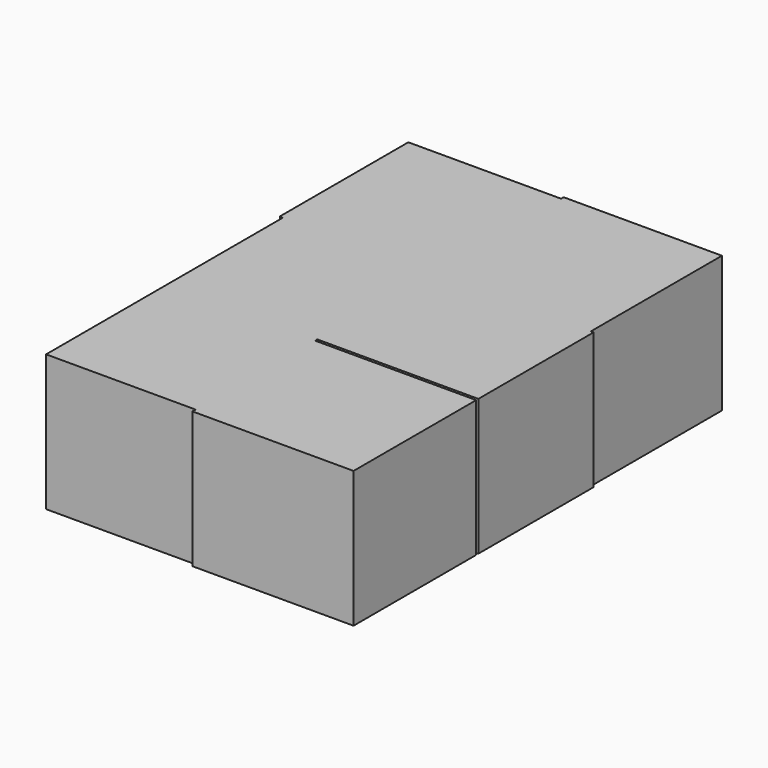
from build123d import *

# Parameters (mm, degrees)
F0_W     = 39.7309437394
F0_H     = 35.8594581485
F0_H_2   = 34.1520495713
F0_W_2   = 39.8523285985
F1_DEPTH = 25.4
F2_W     = 39.7309437394
F2_H     = 34.1520495713
F3_DEPTH = 25.4
F5_W     = 33.1652238965
F5_H     = 31.9460257888
F6_DEPTH = 30.226


with BuildPart() as f1:
    # F0 (on Top) → F1 (new body)
    with BuildSketch(Plane.XY):
        with Locations((-19.8654718697, 17.9297290742)):
            Rectangle(F0_W, F0_H)
        with Locations((-19.8654718697, -17.0760247856)):
            Rectangle(F0_W, F0_H_2)
        with Locations((19.9261642992, 17.9297290742)):
            Rectangle(F0_W_2, F0_H)
    extrude(amount=F1_DEPTH)

    # F2 (on face) → F3 (join)
    with BuildSketch(Plane.XY.offset(25.4)):
        with Locations((-19.8654718697, -17.0760247856)):
            Rectangle(F2_W, F2_H)
    extrude(amount=F3_DEPTH)


with BuildPart() as f6:
    # F5 (on Top) → F6 (new body)
    with BuildSketch(Plane.XY):
        with Locations((-16.5826119483, -15.9730128944)):
            Rectangle(F5_W, F5_H)
        Polygon((-33.1652238965, 0), (0, 0), (0, 35.6270745397), (-33.8673219085, 35.6270745397), (-33.8673219085, 0), align=None)
        Polygon((0, 35.6270745397), (0, 0), (35.113606602, 0), (35.113606602, 36.3328047097), (0, 36.3328047097), align=None)
        Polygon((35.113606602, 0), (0, 0), (0, -31.9460257888), (35.7213914394, -31.9460257888), (35.7213914394, 0), align=None)
        Polygon((0, -32.553806901), (0, -31.9460257888), (-33.1652238965, -31.9460257888), (-33.1652238965, -65.6626299024), (0, -65.6626299024), align=None)
        Polygon((35.7213914394, -32.553806901), (0, -32.553806901), (0, -65.6626299024), (0, -66.5416121483), (35.7213914394, -66.5416121483), align=None)
    extrude(amount=F6_DEPTH)


solid = f6.part
